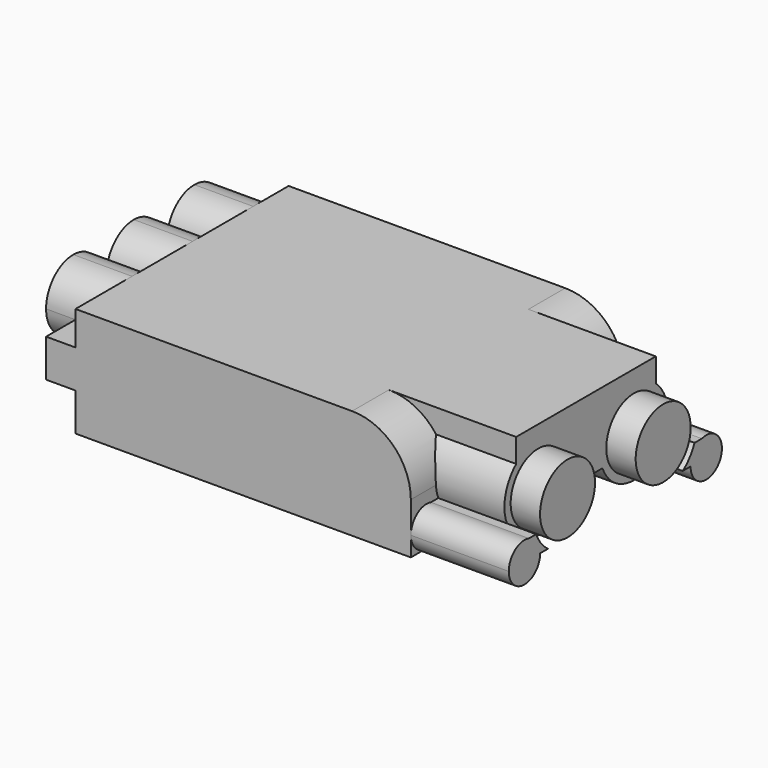
from build123d import *

# Parameters (mm, degrees)
F1_DEPTH  = 17.78
F2_W      = 6.35
F2_H      = 6.1400055
F3_DEPTH  = 9.525
F2_W_2    = 30.48
F4_DEPTH  = 4.7625
F5_R      = 5.5687296145
F6_DEPTH  = 4.7625
F7_DEPTH  = 17.4625
F8_DEPTH  = 25.4
F9_DEPTH  = 15.875
F10_W     = 9.525
F10_H     = 5.08
F10_H_2   = 3.175
F11_DEPTH = 43.18


# Not quite as in the source:
# - a length typed as a fraction of an inch, garbled in the dataset ("3 / 203.2 mm" for 3/8 in), is restored
# - a feature names something its author has since deleted; it is built from what else it names


with BuildPart() as f1:
    # F0 (on Top) → F1 (new body)
    with BuildSketch(Plane.XY):
        Polygon((-39.878, 21.59), (-39.878, 0), (-39.878, -21.59), (39.878, -21.59), (39.878, 0), (39.878, 21.59), align=None)
    extrude(amount=F1_DEPTH)

    # F2 (on face) → F3 (cut)
    with BuildSketch(Plane(origin=(-39.878, 0, 0), x_dir=(0, -1, 0), z_dir=(-1, 0, 0))):
        with Locations((-18.415, 3.07000275)):
            Rectangle(F2_W, F2_H)
        with Locations((18.415, 3.07000275)):
            Rectangle(F2_W, F2_H)
        with BuildLine():
            Line((-21.59, 17.78), (-21.59, 12.28))
            Line((-21.59, 12.28), (-19.9, 12.28))
            ThreePointArc((-19.9, 12.28), (-18.2890872965, 16.1690872965), (-14.4, 17.78))
            Line((-14.4, 17.78), (-21.59, 17.78))
        make_face()
        with BuildLine():
            Line((-2.13, 17.78), (-14.4, 17.78))
            ThreePointArc((-14.4, 17.78), (-10.5109127035, 16.1690872965), (-8.9, 12.28))
            Line((-8.9, 12.28), (-7.63, 12.28))
            ThreePointArc((-7.63, 12.28), (-6.0190872965, 16.1690872965), (-2.13, 17.78))
        make_face()
        with BuildLine():
            Line((15.64, 12.28), (21.59, 12.28))
            Line((21.59, 12.28), (21.59, 17.78))
            Line((21.59, 17.78), (10.14, 17.78))
            ThreePointArc((10.14, 17.78), (14.0290872965, 16.1690872965), (15.64, 12.28))
        make_face()
        with BuildLine():
            Line((10.14, 17.78), (-2.13, 17.78))
            ThreePointArc((-2.13, 17.78), (1.7590872965, 16.1690872965), (3.37, 12.28))
            Line((3.37, 12.28), (4.64, 12.28))
            ThreePointArc((4.64, 12.28), (6.2509127035, 16.1690872965), (10.14, 17.78))
        make_face()
    extrude(amount=-F3_DEPTH, mode=Mode.SUBTRACT)

    # F2 (on face) → F4 (cut)
    with BuildSketch(Plane(origin=(-39.878, 0, 0), x_dir=(0, -1, 0), z_dir=(-1, 0, 0))):
        with Locations((0, 3.07000275)):
            Rectangle(F2_W_2, F2_H)
        with BuildLine():
            Line((-21.59, 12.28), (-21.59, 6.1400055))
            Line((-21.59, 6.1400055), (-15.24, 6.1400055))
            Line((-15.24, 6.1400055), (15.24, 6.1400055))
            Line((15.24, 6.1400055), (21.59, 6.1400055))
            Line((21.59, 6.1400055), (21.59, 12.28))
            Line((21.59, 12.28), (15.64, 12.28))
            ThreePointArc((15.64, 12.28), (10.14, 6.78), (4.64, 12.28))
            Line((4.64, 12.28), (3.37, 12.28))
            ThreePointArc((3.37, 12.28), (-2.13, 6.78), (-7.63, 12.28))
            Line((-7.63, 12.28), (-8.9, 12.28))
            ThreePointArc((-8.9, 12.28), (-14.4, 6.78), (-19.9, 12.28))
            Line((-19.9, 12.28), (-21.59, 12.28))
        make_face()
    extrude(amount=-F4_DEPTH, mode=Mode.SUBTRACT)

    # F5 (on face) → F6 (cut)
    with BuildSketch(Plane.YZ.offset(39.878)):
        with BuildLine():
            Line((14.1410236641, 17.78), (-14.1410236641, 17.78))
            Line((-14.1410236641, 17.78), (-14.1410236641, 13.925705291))
            ThreePointArc((-14.1410236641, 13.925705291), (-8.0583664109, 15.3792022386), (-3.3407865054, 11.2736191532))
            Line((-3.3407865054, 11.2736191532), (3.3407865054, 11.2736191532))
            ThreePointArc((3.3407865054, 11.2736191532), (8.0583664109, 15.3792022386), (14.1410236641, 13.925705291))
            Line((14.1410236641, 13.925705291), (14.1410236641, 17.78))
        make_face()
        with BuildLine():
            ThreePointArc((-14.1410236641, 13.925705291), (-16.3223765845, 10.3766090016), (-16.0373890971, 6.2205090068))
            ThreePointArc((-16.0373890971, 6.2205090068), (-15.0623054432, 4.5248800343), (-13.6467597401, 3.175))
            ThreePointArc((-13.6467597401, 3.175), (-7.7553416056, 2.1900909973), (-3.3407865054, 6.2138400758))
            Line((-3.3407865054, 6.2138400758), (3.3407865054, 6.2138400758))
            ThreePointArc((3.3407865054, 6.2138400758), (7.7553416056, 2.1900909973), (13.6467597401, 3.175))
            ThreePointArc((13.6467597401, 3.175), (15.0623054432, 4.5248800343), (16.0373890971, 6.2205090068))
            ThreePointArc((16.0373890971, 6.2205090068), (16.3223765845, 10.3766090016), (14.1410236641, 13.925705291))
            ThreePointArc((14.1410236641, 13.925705291), (8.0583664109, 15.3792022386), (3.3407865054, 11.2736191532))
            Line((3.3407865054, 11.2736191532), (-3.3407865054, 11.2736191532))
            ThreePointArc((-3.3407865054, 11.2736191532), (-8.0583664109, 15.3792022386), (-14.1410236641, 13.925705291))
        make_face()
        with Locations((-9.6877607201, 8.7437296145)):
            Circle(F5_R, mode=Mode.SUBTRACT)
        with Locations((9.6877607201, 8.7437296145)):
            Circle(F5_R, mode=Mode.SUBTRACT)
    extrude(amount=-F6_DEPTH, mode=Mode.SUBTRACT)

    # F5 (on face) → F7 (cut)
    with BuildSketch(Plane.YZ.offset(39.878)):
        with BuildLine():
            ThreePointArc((-15.24, 3.175), (-16.1699359684, 0.9299359711), (-18.4149999962, 0))
            Line((-18.4149999962, 0), (-12.0420521125, 0))
            Line((-12.0420521125, 0), (18.41500001, 0))
            ThreePointArc((18.41500001, 0), (16.1699359733, 0.9299359662), (15.24, 3.175))
            Line((15.24, 3.175), (13.6467597401, 3.175))
            ThreePointArc((13.6467597401, 3.175), (7.7553416056, 2.1900909973), (3.3407865054, 6.2138400758))
            Line((3.3407865054, 6.2138400758), (-3.3407865054, 6.2138400758))
            ThreePointArc((-3.3407865054, 6.2138400758), (-7.7553416056, 2.1900909973), (-13.6467597401, 3.175))
            Line((-13.6467597401, 3.175), (-15.24, 3.175))
        make_face()
    extrude(amount=-F7_DEPTH, mode=Mode.SUBTRACT)

    # F5 (on face) → F8 (cut)
    with BuildSketch(Plane.YZ.offset(39.878)):
        with BuildLine():
            Line((-21.59, 17.78), (-21.59, 3.175))
            ThreePointArc((-21.59, 3.175), (-20.3164565142, 5.7176537563), (-17.5175035436, 6.2205090068))
            Line((-17.5175035436, 6.2205090068), (-16.0373890971, 6.2205090068))
            ThreePointArc((-16.0373890971, 6.2205090068), (-16.3223765845, 10.3766090016), (-14.1410236641, 13.925705291))
            Line((-14.1410236641, 13.925705291), (-14.1410236641, 17.78))
            Line((-14.1410236641, 17.78), (-21.59, 17.78))
        make_face()
        with BuildLine():
            Line((21.59, 17.78), (14.1410236641, 17.78))
            Line((14.1410236641, 17.78), (14.1410236641, 13.925705291))
            ThreePointArc((14.1410236641, 13.925705291), (16.3223765845, 10.3766090016), (16.0373890971, 6.2205090068))
            Line((16.0373890971, 6.2205090068), (17.5175035436, 6.2205090068))
            ThreePointArc((17.5175035436, 6.2205090068), (20.3164565142, 5.7176537563), (21.59, 3.175))
            Line((21.59, 3.175), (21.59, 17.78))
        make_face()
    extrude(amount=-F8_DEPTH, mode=Mode.SUBTRACT)

    # F5 (on face) → F9 (cut)
    with BuildSketch(Plane.YZ.offset(39.878)):
        with BuildLine():
            Line((-21.59, 3.175), (-21.59, 0))
            Line((-21.59, 0), (-18.4149999962, 0))
            ThreePointArc((-18.4149999962, 0), (-20.6600640289, 0.9299359684), (-21.59, 3.175))
        make_face()
        with BuildLine():
            ThreePointArc((-15.24, 3.175), (-16.1699359684, 0.9299359711), (-18.4149999962, 0))
            Line((-18.4149999962, 0), (-12.0420521125, 0))
            Line((-12.0420521125, 0), (18.41500001, 0))
            ThreePointArc((18.41500001, 0), (16.1699359733, 0.9299359662), (15.24, 3.175))
            Line((15.24, 3.175), (13.6467597401, 3.175))
            ThreePointArc((13.6467597401, 3.175), (7.7553416056, 2.1900909973), (3.3407865054, 6.2138400758))
            Line((3.3407865054, 6.2138400758), (-3.3407865054, 6.2138400758))
            ThreePointArc((-3.3407865054, 6.2138400758), (-7.7553416056, 2.1900909973), (-13.6467597401, 3.175))
            Line((-13.6467597401, 3.175), (-15.24, 3.175))
        make_face()
        with BuildLine():
            ThreePointArc((21.59, 3.175), (20.6600640338, 0.9299359733), (18.41500001, 0))
            Line((18.41500001, 0), (21.59, 0))
            Line((21.59, 0), (21.59, 3.175))
        make_face()
    extrude(amount=-F9_DEPTH, mode=Mode.SUBTRACT)

    # F10 (on face) → F11 (join)
    with BuildSketch(Plane.XZ.offset(21.59)):
        with BuildLine():
            ThreePointArc((24.003, 8.255), (21.2131920908, 14.9901920908), (14.478, 17.78))
            Line((14.478, 17.78), (14.478, 8.255))
            Line((14.478, 8.255), (24.003, 8.255))
        make_face()
        with Locations((19.2405, 5.715)):
            Rectangle(F10_W, F10_H)
        with Locations((19.2405, 1.5875)):
            Rectangle(F10_W, F10_H_2)
    extrude(amount=-F11_DEPTH)


solid = f1.part
